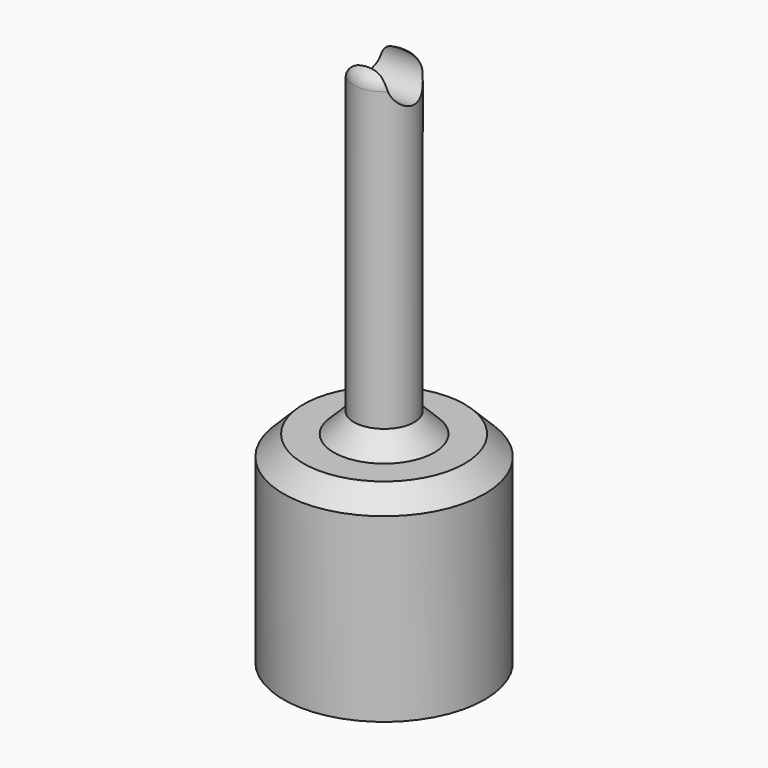
from build123d import *

# Parameters (mm, degrees)
F0_R        = 5
F1_DEPTH    = 10
F2_R        = 1.5
F3_DEPTH    = 16
F7_SIZE     = 1
F8_DEPTH    = 12.5
F9_T2_ANGLE = 245.2760469103
F9_T4_ANGLE = 245.2760469103


# Not quite as in the source:
# - a fillet or chamfer that OpenCascade refuses, or shapes differently, is made with other operations: its cross-section is extruded or revolved along the edge and cut away or added


with BuildPart() as f1:
    # F0 (on Top) → F1 (new body)
    with BuildSketch(Plane.XY):
        Circle(F0_R)
    extrude(amount=F1_DEPTH)

    # F2 (on face) → F3 (join)
    with BuildSketch(Plane.XY.offset(10)):
        Circle(F2_R)
    extrude(amount=F3_DEPTH)

    # F4 (on Right) → F5 (revolve)
    with BuildSketch(Plane.YZ):
        with BuildLine():
            ThreePointArc((1.5, 26), (0, 27.5), (-1.5, 26))
            Line((-1.5, 26), (1.5, 26))
        make_face()
    revolve(axis=Axis((0, 0, 26), (0, 1, 0)))

    # F7
    f7_edges = [f1.edges().sort_by_distance(p)[0] for p in [
        (-5, 0, 10),
        (-1.5, 0, 10),
    ]]
    chamfer(f7_edges, length=F7_SIZE)

    # F6 (on Right) → F8 (cut, symmetric)
    with BuildSketch(Plane.YZ):
        with BuildLine():
            Line((-1.4142135624, 26.5), (-0.9797958971, 26.5))
            ThreePointArc((-0.9797958971, 26.5), (0, 24.9), (0.9797958971, 26.5))
            Line((0.9797958971, 26.5), (1.4142135624, 26.5))
            ThreePointArc((1.4142135624, 26.5), (0, 27.5), (-1.4142135624, 26.5))
        make_face()
    extrude(amount=F8_DEPTH, both=True, mode=Mode.SUBTRACT)

    # F9: fillet of radius 0.75 on 2 edges, made by hand

    # F9_s1 → F9_t2 (revolve, cut)
    with BuildSketch(Plane(origin=(0, 0, 0), x_dir=(0, 0, 1), z_dir=(0.5393297468, -0.8420946646, 0))):
        with BuildLine():
            ThreePointArc((25.75, 1.5), (26.2803300859, 1.2803300859), (26.5, 0.75))
            Line((26.5, 0.75), (26.575, 0.75))
            Line((26.575, 0.75), (26.575, 1.4142135624))
            Line((26.575, 1.4142135624), (26.525, 1.4849242405))
            ThreePointArc((26.525, 1.4849242405), (26, 1.575), (25.75, 1.575))
            Line((25.75, 1.575), (25.75, 1.5))
        make_face()
    revolve(axis=Axis((0, 0, 26.5), (0, 0, -1)), revolution_arc=F9_T2_ANGLE, mode=Mode.SUBTRACT)

    # F9_s3 → F9_t4 (revolve, cut)
    with BuildSketch(Plane(origin=(0, 0, 0), x_dir=(0, 0, 1), z_dir=(-0.5393297468, 0.8420946646, 0))):
        with BuildLine():
            ThreePointArc((25.75, 1.5), (26.2803300859, 1.2803300859), (26.5, 0.75))
            Line((26.5, 0.75), (26.575, 0.75))
            Line((26.575, 0.75), (26.575, 1.4142135624))
            Line((26.575, 1.4142135624), (26.525, 1.4849242405))
            ThreePointArc((26.525, 1.4849242405), (26, 1.575), (25.75, 1.575))
            Line((25.75, 1.575), (25.75, 1.5))
        make_face()
    revolve(axis=Axis((0, 0, 26.5), (0, 0, -1)), revolution_arc=F9_T4_ANGLE, mode=Mode.SUBTRACT)


solid = f1.part
